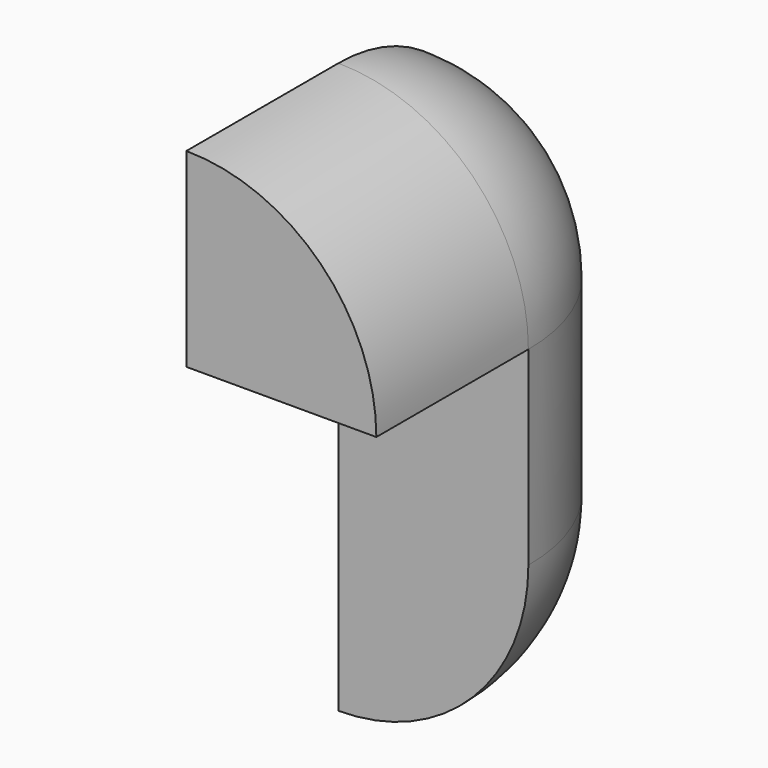
from build123d import *

# Parameters (mm, degrees)
F0_W     = 25.4
F0_H     = 25.4
F1_DEPTH = 76.2
F2_W     = 25.4
F2_H     = 25.4
F3_DEPTH = 25.4
F4_R     = 25.39999


# Not quite as in the source:
# - a fillet or chamfer is up to 0.001 mm smaller than in the source, because OpenCascade refuses the exact size


with BuildPart() as f1:
    # F0 (on Top) → F1 (new body)
    with BuildSketch(Plane.XY):
        with Locations((12.7, 12.7)):
            Rectangle(F0_W, F0_H)
    extrude(amount=F1_DEPTH)

    # F2 (on face) → F3 (join)
    with BuildSketch(Plane.XZ):
        with Locations((12.7, 63.5)):
            Rectangle(F2_W, F2_H)
    extrude(amount=F3_DEPTH)

    # F4 (radius 25.4 in the source; OpenCascade refuses exactly that, so slightly less here)
    f4_edges = [f1.edges().sort_by_distance(p)[0] for p in [
        (12.7, 25.4, 0),
        (25.4, 12.7, 0),
        (25.4, 25.4, 38.1),
        (25.4, 0, 76.2),
        (12.7, 25.4, 76.2),
    ]]
    fillet(f4_edges, radius=F4_R)


solid = f1.part
